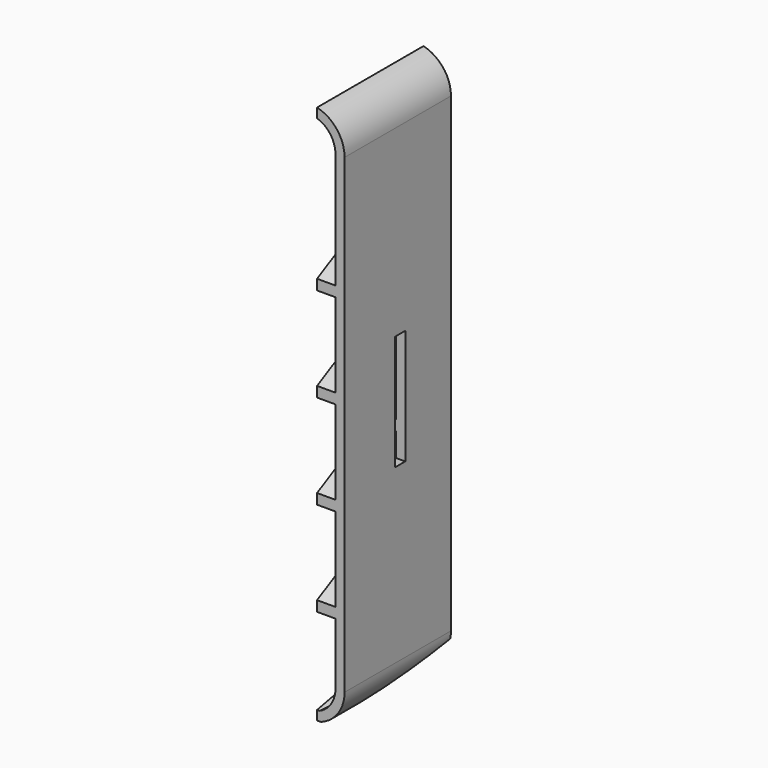
from build123d import *

# Parameters (mm, degrees)
F1_DEPTH    = 37
F2_T1_DEPTH = 342.8505669038
F3_T        = -2.54
F4_W        = 125.55387271
F4_H        = 111.9176980871
F5_DEPTH    = 25.4
F6_R        = 3.175
F7_DEPTH    = 19.05
F9_DEPTH    = 142.24
F10_W       = 3.5
F10_H       = 32
F11_DEPTH   = 5
F12_W       = 142.5411626697
F12_H       = 154.7065079212
F13_DEPTH   = 37.001


# Not quite as in the source:
# - a fillet or chamfer that OpenCascade refuses, or shapes differently, is made with other operations: its cross-section is extruded or revolved along the edge and cut away or added


with BuildPart() as f1:
    # F0 (on Front) → F1 (new body)
    with BuildSketch(Plane.XZ):
        with BuildLine():
            Line((62.5, 75.5), (-72.5, 75.5))
            Line((-72.5, 75.5), (-72.5, -75.5))
            Line((-72.5, -75.5), (62.5, -75.5))
            ThreePointArc((62.5, -75.5), (69.5710678119, -72.5710678119), (72.5, -65.5))
            Line((72.5, -65.5), (72.5, 65.5))
            ThreePointArc((72.5, 65.5), (69.5710678119, 72.5710678119), (62.5, 75.5))
        make_face()
    extrude(amount=F1_DEPTH)

    # F2: chamfer of 40 x 8 on 1 edges, made by hand

    # F2_s2 → F2_t1 (cut)
    with BuildSketch(Plane.YZ.offset(-176.4252834519)):
        Polygon((-40, -75.5), (0, -67.5), (0, -75.5), align=None)
    extrude(amount=F2_T1_DEPTH, mode=Mode.SUBTRACT)

    # F3
    f3_openings = [f1.faces().sort_by_distance(p)[0] for p in [
        (-0.123954, -37, 0.284541),
    ]]
    offset(amount=F3_T, openings=f3_openings)

    # F4 (on face) → F5 (cut)
    with BuildSketch(Plane.XZ.offset(2.54)):
        with Locations((-0.276936355, 9.5411509565)):
            Rectangle(F4_W, F4_H)
    extrude(amount=-F5_DEPTH, mode=Mode.SUBTRACT)

    # F6 (on face) → F7 (cut)
    with BuildSketch(Plane(origin=(-72.5, 0, 0), x_dir=(0, -1, 0), z_dir=(-1, 0, 0))):
        with Locations((21.3561020792, 0)):
            Circle(F6_R)
        with Locations((21.3561020792, 35)):
            Circle(F6_R)
        with Locations((21.3561020792, -30)):
            Circle(F6_R)
    extrude(amount=-F7_DEPTH, mode=Mode.SUBTRACT)

    # F8 (on face) → F9 (join)
    with BuildSketch(Plane(origin=(69.96, 0, 0), x_dir=(0, -1, 0), z_dir=(-1, 0, 0))):
        Polygon((0, -28.8742875891), (37, -48.2893098931), (37, -45.4208615419), (0, -26.005839238), align=None)
        Polygon((0, -2.637839238), (37, -22.0528615419), (37, -19.1844131908), (0, 0.2306091132), align=None)
        Polygon((0, 23.5986091132), (37, 4.1835868092), (37, 7.0520351604), (0, 26.4670574643), align=None)
        Polygon((0, 49.8350574643), (37, 30.4200351604), (37, 33.2884835115), (0, 52.7035058155), align=None)
    extrude(amount=F9_DEPTH)

    # F10 (on face) → F11 (cut)
    with BuildSketch(Plane.YZ.offset(72.5)):
        with Locations((-17.6429149747, -1.5458973408)):
            Rectangle(F10_W, F10_H)
    extrude(amount=-F11_DEPTH, mode=Mode.SUBTRACT)

    # F12 (on face) → F13 (cut, through all)
    with BuildSketch(Plane.XZ.offset(37)):
        with Locations((-6.4269788563, 0.7590651512)):
            Rectangle(F12_W, F12_H)
    extrude(amount=-F13_DEPTH, mode=Mode.SUBTRACT)


solid = f1.part
